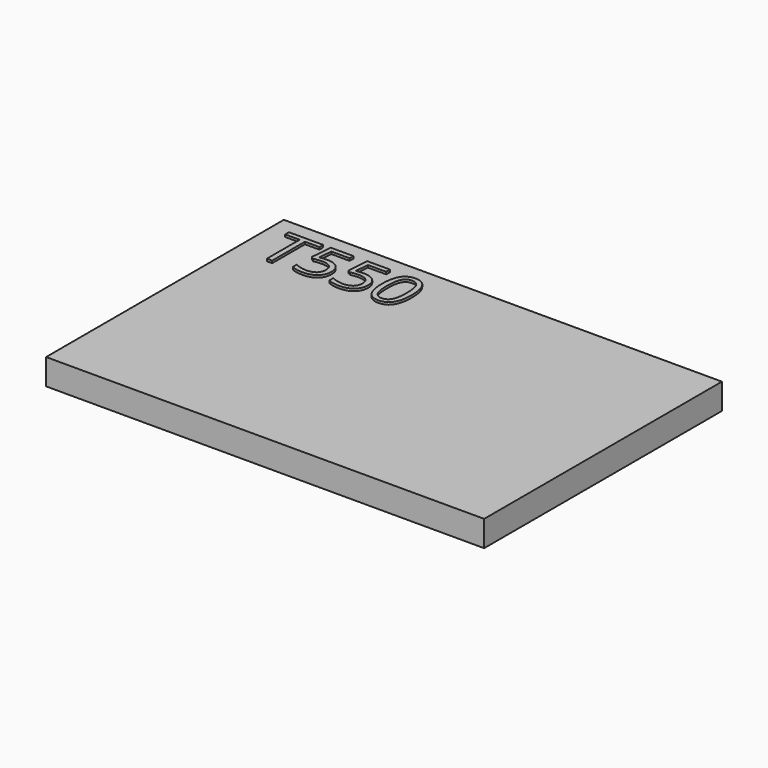
from build123d import *

# Parameters (mm, degrees)
F0_W         = 380.6
F0_H         = 258.2
F1_DEPTH     = 22.45
F2_TEXT_SIZE = 55.5555555556
F3_DEPTH     = 2


# Not quite as in the source:
# - Text() gives the source's letters only with a copy of the font that has no kerning and outlines rounded to 1/6400 em; it was checked with that copy


with BuildPart() as f1:
    # F0 (on Top) → F1 (new body)
    with BuildSketch(Plane.XY):
        with Locations((4.3076434314, -21.3974882992)):
            Rectangle(F0_W, F0_H)
    extrude(amount=F1_DEPTH)

    # F2 (on face) → F3 (join)
    with BuildSketch(Plane.XY.offset(22.45)):
        with Locations((-169.9590253531, 52.9430953035)):
            Text('T550', F2_TEXT_SIZE, font='Open Sans', text_align=(TextAlign.LEFT, TextAlign.BOTTOM))
    extrude(amount=F3_DEPTH)


solid = f1.part
